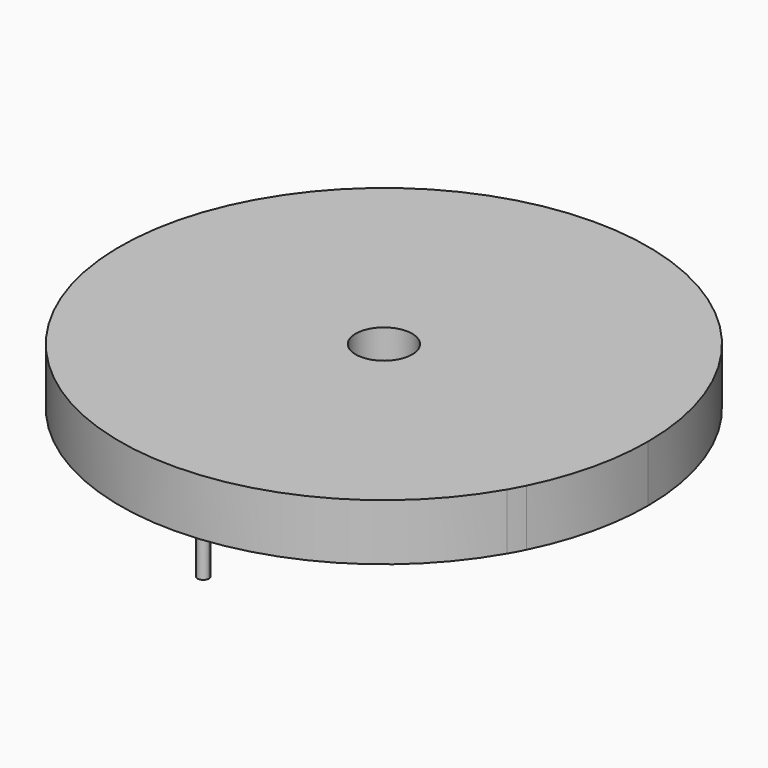
from build123d import *

# Parameters (mm, degrees)
F1_DEPTH = 12.7
F2_DEPTH = 12.7


with BuildPart() as f1:
    # F0 (on Top) → F1 (new body)
    with BuildSketch(Plane.XY):
        with BuildLine():
            Line((1.27, 0), (0, 0))
            Line((0, 0), (0, 1.27))
            ThreePointArc((0, 1.27), (-0.8980256121, -0.8980256121), (1.27, 0))
        make_face()
        with BuildLine():
            Line((0, 1.27), (0, 0))
            Line((0, 0), (1.27, 0))
            ThreePointArc((1.27, 0), (0.8980256121, 0.8980256121), (0, 1.27))
        make_face()
        with BuildLine():
            ThreePointArc((1.27, 0), (-0.8980256121, -0.8980256121), (0, 1.27))
            Line((0, 1.27), (0, 16.51))
            ThreePointArc((0, 16.51), (-18.5637162853, 21.9695900536), (-31.2160717781, 36.6098286569))
            ThreePointArc((-31.2160717781, 36.6098286569), (-42.6516552572, 31.3045995485), (-53.2117304222, 24.4196276597))
            ThreePointArc((-53.2117304222, 24.4196276597), (-16.5828563916, -6.2300023956), (30.7696652459, 0))
            Line((30.7696652459, 0), (1.27, 0))
        make_face()
        with BuildLine():
            Line((0, 16.51), (0, 1.27))
            ThreePointArc((0, 1.27), (0.8980256121, 0.8980256121), (1.27, 0))
            Line((1.27, 0), (30.7696652459, 0))
            ThreePointArc((30.7696652459, 0), (42.4352015878, 9.2468296571), (51.4349999952, 21.103988907))
            Line((51.4349999952, 21.103988907), (29.6960110958, 33.655))
            ThreePointArc((29.6960110958, 33.655), (17.145, 21.1039889042), (0, 16.51))
        make_face()
        with BuildLine():
            ThreePointArc((-31.2160717781, 36.6098286569), (-18.5637162853, 21.9695900536), (0, 16.51))
            Line((0, 16.51), (0, 42.3333333333))
            ThreePointArc((0, 42.3333333333), (-15.8682201509, 40.8906294723), (-31.2160717781, 36.6098286569))
        make_face()
        with BuildLine():
            Line((0, 42.3333333333), (0, 16.51))
            ThreePointArc((0, 16.51), (17.145, 21.1039889042), (29.6960110958, 33.655))
            Line((29.6960110958, 33.655), (17.8245764663, 40.508975979))
            ThreePointArc((17.8245764663, 40.508975979), (8.9588476653, 41.8760557513), (0, 42.3333333333))
        make_face()
        with BuildLine():
            ThreePointArc((-31.2160717781, 36.6098286569), (-15.8682201509, 40.8906294723), (0, 42.3333333333))
            Line((0, 42.3333333333), (0, 44.45))
            ThreePointArc((0, 44.45), (-4.4901280605, 55.2901280605), (6.35, 50.8))
            ThreePointArc((6.35, 50.8), (6.1336289969, 49.1564990636), (5.499261314, 47.625))
            Line((5.499261314, 47.625), (17.8245764663, 40.508975979))
            ThreePointArc((17.8245764663, 40.508975979), (24.5977058385, 38.8251673187), (31.2160717781, 36.6098286569))
            ThreePointArc((31.2160717781, 36.6098286569), (33.5127080469, 43.5403512919), (34.29, 50.8))
            ThreePointArc((34.29, 50.8), (-7.2596487081, 84.3127080469), (-31.2160717781, 36.6098286569))
        make_face()
        with BuildLine():
            Line((0, 44.45), (0, 42.3333333333))
            ThreePointArc((0, 42.3333333333), (8.9588476653, 41.8760557513), (17.8245764663, 40.508975979))
            Line((17.8245764663, 40.508975979), (5.499261314, 47.625))
            ThreePointArc((5.499261314, 47.625), (3.175, 45.300738686), (0, 44.45))
        make_face()
        with BuildLine():
            ThreePointArc((-53.2117304222, 24.4196276597), (-42.6516552572, 31.3045995485), (-31.2160717781, 36.6098286569))
            ThreePointArc((-31.2160717781, 36.6098286569), (-7.2596487081, 84.3127080469), (34.29, 50.8))
            ThreePointArc((34.29, 50.8), (33.5127080469, 43.5403512919), (31.2160717781, 36.6098286569))
            ThreePointArc((31.2160717781, 36.6098286569), (42.6516552572, 31.3045995485), (53.2117304222, 24.4196276597))
            ThreePointArc((53.2117304222, 24.4196276597), (57.8263113692, 37.2526750694), (59.392022186, 50.8))
            ThreePointArc((59.392022186, 50.8), (-13.5473249306, 108.6263113692), (-53.2117304222, 24.4196276597))
        make_face()
        with BuildLine():
            ThreePointArc((31.2160717781, 36.6098286569), (30.4918548649, 35.1139907276), (29.6960110958, 33.655))
            Line((29.6960110958, 33.655), (51.4349999952, 21.103988907))
            ThreePointArc((51.4349999952, 21.103988907), (52.3496218883, 22.7477382821), (53.2117304222, 24.4196276597))
            ThreePointArc((53.2117304222, 24.4196276597), (42.6516552572, 31.3045995485), (31.2160717781, 36.6098286569))
        make_face()
        with BuildLine():
            Line((17.8245764663, 40.508975979), (29.6960110958, 33.655))
            ThreePointArc((29.6960110958, 33.655), (30.4918548649, 35.1139907276), (31.2160717781, 36.6098286569))
            ThreePointArc((31.2160717781, 36.6098286569), (24.5977058385, 38.8251673187), (17.8245764663, 40.508975979))
        make_face()
    extrude(amount=F1_DEPTH)

    # F0 (on Top) → F2 (join)
    with BuildSketch(Plane.XY):
        with BuildLine():
            Line((0, 1.27), (0, 0))
            Line((0, 0), (1.27, 0))
            ThreePointArc((1.27, 0), (0.8980256121, 0.8980256121), (0, 1.27))
        make_face()
        with BuildLine():
            Line((1.27, 0), (0, 0))
            Line((0, 0), (0, 1.27))
            ThreePointArc((0, 1.27), (-0.8980256121, -0.8980256121), (1.27, 0))
        make_face()
        with BuildLine():
            ThreePointArc((-31.2160717781, 36.6098286569), (-15.8682201509, 40.8906294723), (0, 42.3333333333))
            Line((0, 42.3333333333), (0, 44.45))
            ThreePointArc((0, 44.45), (-4.4901280605, 55.2901280605), (6.35, 50.8))
            ThreePointArc((6.35, 50.8), (6.1336289969, 49.1564990636), (5.499261314, 47.625))
            Line((5.499261314, 47.625), (17.8245764663, 40.508975979))
            ThreePointArc((17.8245764663, 40.508975979), (24.5977058385, 38.8251673187), (31.2160717781, 36.6098286569))
            ThreePointArc((31.2160717781, 36.6098286569), (33.5127080469, 43.5403512919), (34.29, 50.8))
            ThreePointArc((34.29, 50.8), (-7.2596487081, 84.3127080469), (-31.2160717781, 36.6098286569))
        make_face()
        with BuildLine():
            Line((0, 44.45), (0, 42.3333333333))
            ThreePointArc((0, 42.3333333333), (8.9588476653, 41.8760557513), (17.8245764663, 40.508975979))
            Line((17.8245764663, 40.508975979), (5.499261314, 47.625))
            ThreePointArc((5.499261314, 47.625), (3.175, 45.300738686), (0, 44.45))
        make_face()
    extrude(amount=-F2_DEPTH)


solid = f1.part
